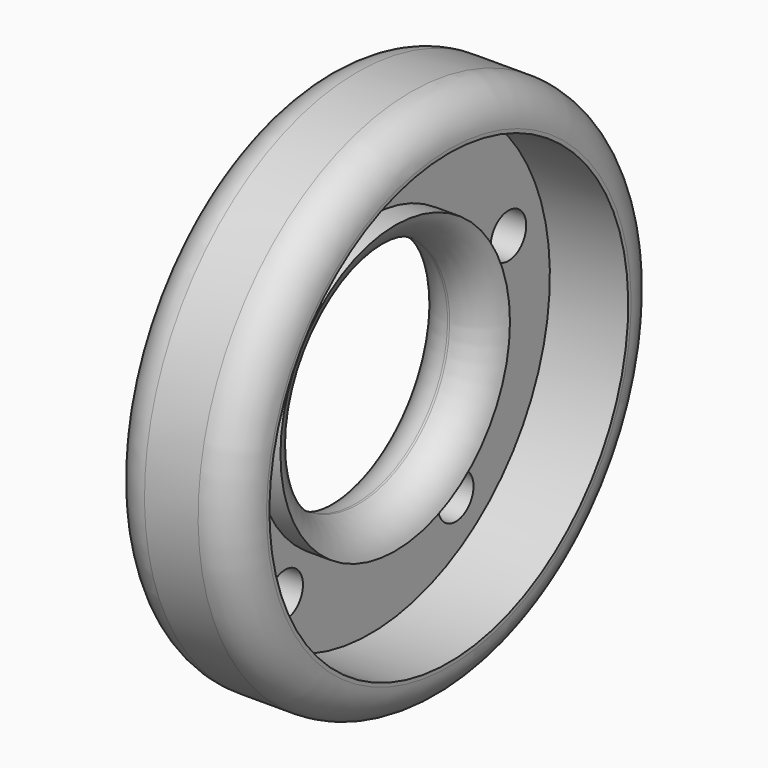
from build123d import *

# Parameters (mm, degrees)
F2_R     = 2.9212519553
F3_DEPTH = 25


# Not quite as in the source:
# - a fillet or chamfer that OpenCascade refuses, or shapes differently, is made with other operations: its cross-section is extruded or revolved along the edge and cut away or added


with BuildPart() as f1:
    # F0 (on Front) → F1 (revolve)
    with BuildSketch(Plane.XZ):
        Polygon((0, 18.8674032688), (0, 15.0357997045), (10, 15.0357997045), (10, 18.8674032688), (6.7462138832, 18.8674032688), (6.7462138832, 29.4962655753), (17.0517656952, 29.4962655753), (17.0517656952, 34.9722243845), (0, 34.9722243845), (0, 29.4962655753), (2.411958063, 29.4962655753), (2.411958063, 18.8674032688), align=None)
    revolve(axis=Axis((6.3371746801, 0, 0), (1, 0, 0)))

    # F2 (on face) → F3 (cut)
    with BuildSketch(Plane(origin=(2.411958063, 0, 0), x_dir=(0, -1, 0), z_dir=(-1, 0, 0))):
        with Locations((-22.6866142127, 7.3713277985)):
            Circle(F2_R)
        with Locations((0, 23.8541178405)):
            Circle(F2_R)
        with Locations((22.6866142127, 7.3713277985)):
            Circle(F2_R)
        with Locations((14.0210986731, -19.2983867188)):
            Circle(F2_R)
        with Locations((-14.0210986731, -19.2983867188)):
            Circle(F2_R)
    extrude(amount=-F3_DEPTH, mode=Mode.SUBTRACT)

    # F4: fillet of radius 5 on 4 edges, made by hand

    # F4_s1 → F4_t2 (revolve, cut)
    with BuildSketch(Plane.XZ):
        with BuildLine():
            ThreePointArc((0, 29.9722243845), (1.4644660941, 33.5077582905), (5, 34.9722243845))
            Line((5, 34.9722243845), (5, 35.0722243845))
            Line((5, 35.0722243845), (-0.1, 35.0722243845))
            Line((-0.1, 35.0722243845), (-0.1, 29.9722243845))
            Line((-0.1, 29.9722243845), (0, 29.9722243845))
        make_face()
    revolve(axis=Axis((0, 0, 0), (1, 0, 0)), mode=Mode.SUBTRACT)

    # F4_s3 → F4_t4 (revolve, cut)
    with BuildSketch(Plane.XZ):
        with BuildLine():
            ThreePointArc((0, 18.8674032688), (1.7665712524, 16.1088427288), (4.8615686531, 15.0357997045))
            Line((4.8615686531, 15.0357997045), (4.8615686531, 14.9357997045))
            Line((4.8615686531, 14.9357997045), (0, 14.9357997045))
            Line((0, 14.9357997045), (-0.1, 15.0357997045))
            ThreePointArc((-0.1, 15.0357997045), (-0.1, 16.9516014867), (-0.0972313731, 18.8440353401))
            Line((-0.0972313731, 18.8440353401), (0, 18.8674032688))
        make_face()
    revolve(axis=Axis((0, 0, 0), (1, 0, 0)), mode=Mode.SUBTRACT)

    # F4_s5 → F4_t6 (revolve, cut)
    with BuildSketch(Plane.XZ):
        with BuildLine():
            ThreePointArc((12.0517656952, 34.9722243845), (15.5872996011, 33.5077582905), (17.0517656952, 29.9722243845))
            Line((17.0517656952, 29.9722243845), (17.1517656952, 29.9722243845))
            Line((17.1517656952, 29.9722243845), (17.1517656952, 35.0722243845))
            Line((17.1517656952, 35.0722243845), (12.0517656952, 35.0722243845))
            Line((12.0517656952, 35.0722243845), (12.0517656952, 34.9722243845))
        make_face()
    revolve(axis=Axis((17.0517656952, 0, 0), (1, 0, 0)), mode=Mode.SUBTRACT)

    # F4_s7 → F4_t8 (revolve, cut)
    with BuildSketch(Plane.XZ):
        with BuildLine():
            ThreePointArc((5.1384313469, 15.0357997045), (8.2334287476, 16.1088427288), (10, 18.8674032688))
            Line((10, 18.8674032688), (10.0972313731, 18.8440353401))
            ThreePointArc((10.0972313731, 18.8440353401), (10.1, 16.9516014867), (10.1, 15.0357997045))
            Line((10.1, 15.0357997045), (10, 14.9357997045))
            Line((10, 14.9357997045), (5.1384313469, 14.9357997045))
            Line((5.1384313469, 14.9357997045), (5.1384313469, 15.0357997045))
        make_face()
    revolve(axis=Axis((10, 0, 0), (1, 0, 0)), mode=Mode.SUBTRACT)


solid = f1.part
